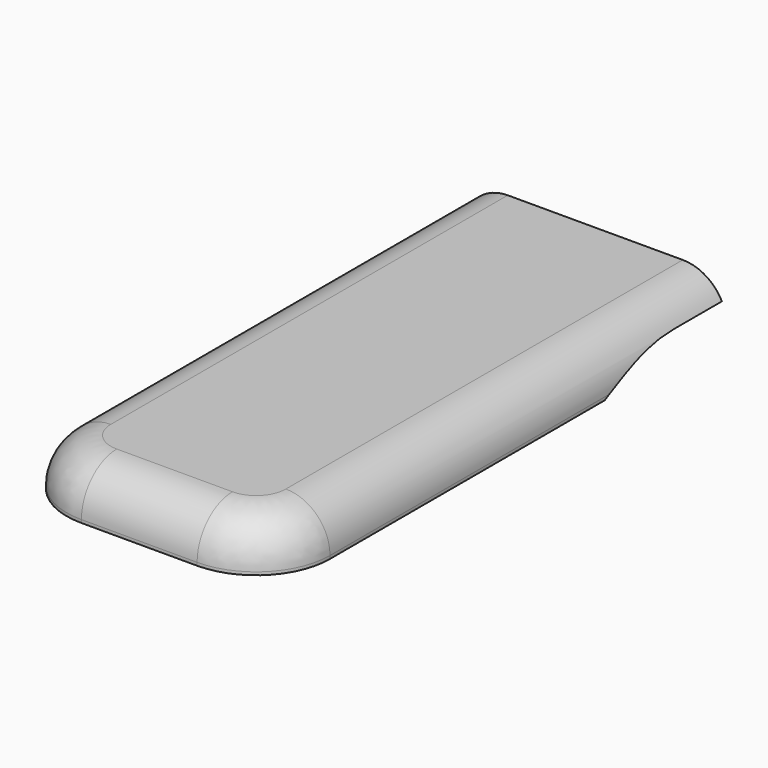
from build123d import *

# Parameters (mm, degrees)
F1_DEPTH      = 95
F3_DEPTH      = 68
F4_W          = 9.75
F4_H          = 1
F5_ANGLE      = 90
F6_W          = 9.75
F6_H          = 1
F7_DEPTH      = 19
F8_DEPTH      = 19
F12_DEPTH     = 86.5
F15_TEXT_SIZE = 7.0614196396
F16_DEPTH     = 0.5


# Not quite as in the source:
# - Text() gives the source's letters only with a copy of the font that has no kerning and outlines rounded to 1/6400 em; it was checked with that copy


with BuildPart() as f1:
    # F0 (on Front) → F1 (new body)
    with BuildSketch(Plane.XZ):
        with BuildLine():
            Line((0, 15.5), (-28.75, 15.5))
            ThreePointArc((-28.75, 15.5), (-39.0030483272, 11.2530483272), (-43.25, 1))
            Line((-43.25, 1), (-43.25, 0))
            Line((-43.25, 0), (-42.25, 0))
            Line((-42.25, 0), (-40.75, 0))
            Line((-40.75, 0), (-40.75, 1))
            Line((-40.75, 1), (-42.25, 1))
            ThreePointArc((-42.25, 1), (-38.295941546, 10.545941546), (-28.75, 14.5))
            Line((-28.75, 14.5), (0, 14.5))
            Line((0, 14.5), (0, 15.5))
        make_face()
    extrude(amount=F1_DEPTH)

    # F2 (on face) → F3 (join)
    with BuildSketch(Plane(origin=(0, 0, 0), x_dir=(-1, 0, 0), z_dir=(0, 1, 0))):
        with BuildLine():
            ThreePointArc((28.75, 14.5), (38.295941546, 10.545941546), (42.25, 1))
            Line((42.25, 1), (42.25, 0))
            Line((42.25, 0), (43.25, 0))
            Line((43.25, 0), (43.25, 1))
            ThreePointArc((43.25, 1), (39.0030483272, 11.2530483272), (28.75, 15.5))
            Line((28.75, 15.5), (0, 15.5))
            Line((0, 15.5), (0, 14.5))
            Line((0, 14.5), (28.75, 14.5))
        make_face()
    extrude(amount=F3_DEPTH)

    # F4 (on face) → F5 (revolve)
    with BuildSketch(Plane.XZ.offset(95)):
        with BuildLine():
            Line((-42.25, 0), (-42.25, 1))
            ThreePointArc((-42.25, 1), (-38.295941546, 10.545941546), (-28.75, 14.5))
            Line((-28.75, 14.5), (-28.75, 15.5))
            ThreePointArc((-28.75, 15.5), (-39.0030483272, 11.2530483272), (-43.25, 1))
            Line((-43.25, 1), (-43.25, 0))
            Line((-43.25, 0), (-42.25, 0))
        make_face()
        with Locations((-23.875, 15)):
            Rectangle(F4_W, F4_H)
    revolve(axis=Axis((-19, -95, 15), (0, 0, 1)), revolution_arc=F5_ANGLE)

    # F6 (on face) → F7 (join, through all)
    with BuildSketch(Plane.YZ.offset(-19)):
        with Locations((-99.875, 15)):
            Rectangle(F6_W, F6_H)
    extrude(amount=F7_DEPTH)

    # F8 (add, through all): a face of the model
    f8_faces = [f1.faces().sort_by_distance(p)[0] for p in [
        (-19, -114.852965017, 11.102965017),
    ]]
    extrude(f8_faces, amount=F8_DEPTH)

    # F9: F1 across plane


with BuildPart() as f1_1:
    add(f1.part)
    add(f1.part.mirror(Plane.YZ))

    # F11 (on face) → F12 (cut, through all)
    with BuildSketch(Plane.YZ.offset(43.25)):
        with BuildLine():
            ThreePointArc((48, 7.7), (32.4256482896, 5.7446571325), (17.8180231795, 0))
            Line((17.8180231795, 0), (68, 0))
            Line((68, 0), (68, 1))
            Line((68, 1), (68, 7.7))
            Line((68, 7.7), (48, 7.7))
        make_face()
    extrude(amount=-F12_DEPTH, mode=Mode.SUBTRACT)


with BuildPart() as f13_1:
    # F13: copy of F1
    add(f1_1.part.moved(Location((180, 0, 0))))


with BuildPart() as f1_2:
    add(f1_1.part)

    # F15 (on face) → F16 (cut)
    with BuildSketch(Plane(origin=(0, 0, 14.5), x_dir=(1, 0, 0), z_dir=(0, 0, -1))):
        with Locations(Location((2.5421110702, -24), (0, 0, 90))):
            Text('ashlynn.crisp@pcc.edu', F15_TEXT_SIZE, font='Open Sans', text_align=(TextAlign.LEFT, TextAlign.BOTTOM))
    extrude(amount=-F16_DEPTH, mode=Mode.SUBTRACT)


solid = f1_2.part
